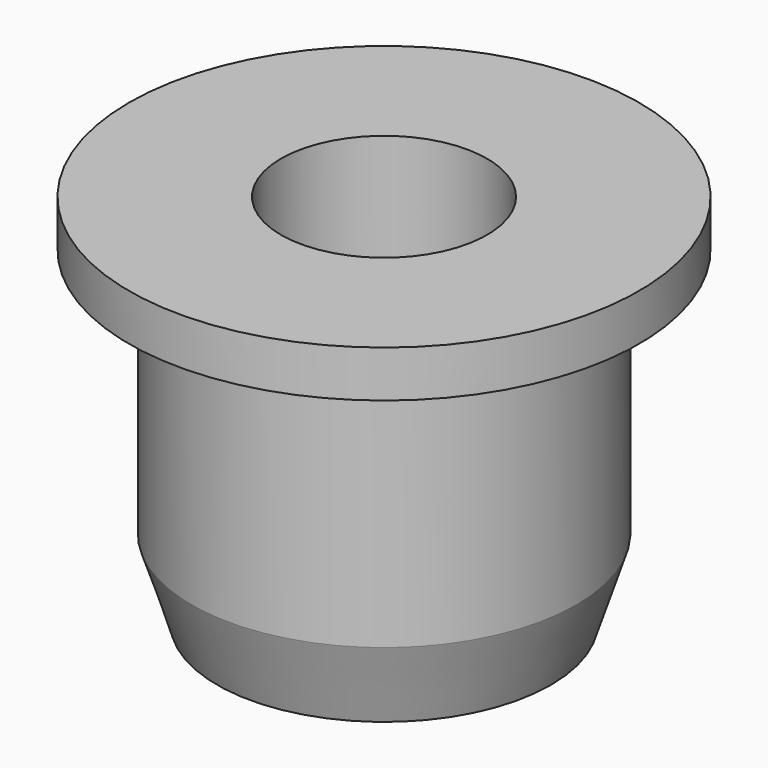
from build123d import *


# Not quite as in the source:
# - a feature names something its author has since deleted; it is built from what else it names


with BuildPart() as f1:
    # F0 (on Front) → F1 (revolve)
    with BuildSketch(Plane.XZ):
        Polygon((-13.335, 48.5521), (-32.97555, 48.5521), (-32.97555, 42.5196), (-24.8666, 42.5196), (-24.8666, 10.1854), (-21.5773, 0), (-13.335, 0), align=None)
    revolve(axis=Axis((0, 0, 24.27605), (0, 0, 1)))


solid = f1.part
